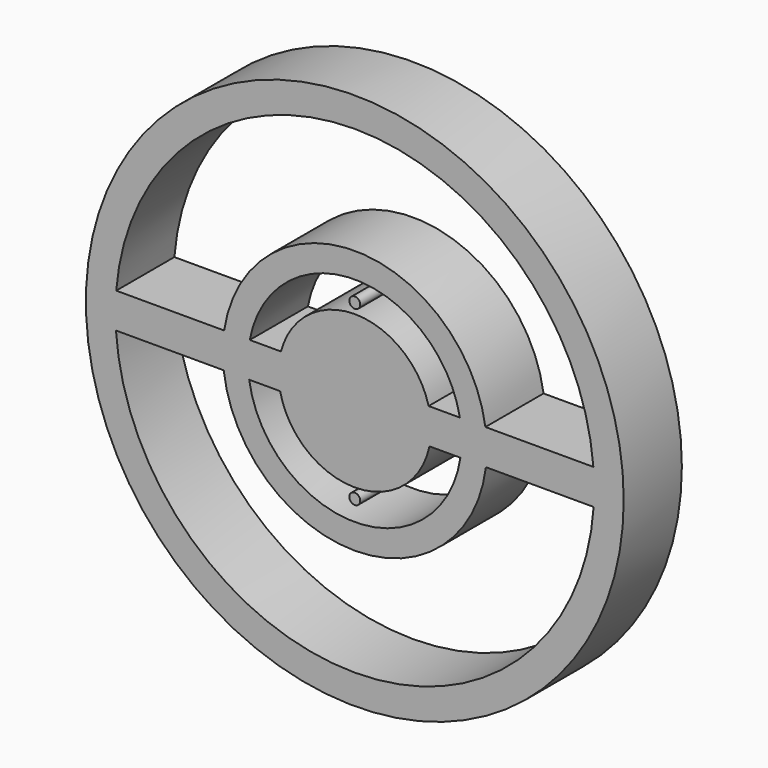
from build123d import *

# Parameters (mm, degrees)
F0_R     = 93.98
F0_W     = 9.525
F0_H     = 25.4
F1_DEPTH = 25.4
F0_R_2   = 1.905


# Not quite as in the source:
# - a feature of the source that left no trace in its solid (it failed there, or was rolled back) is left out


with BuildPart() as f1:
    # F0 (on Front) → F1 (new body)
    with BuildSketch(Plane.XZ):
        Circle(F0_R)
        with BuildLine():
            ThreePointArc((-45.8102837042, -5.5278504869), (0, -46.1425966333), (45.8102837042, -5.5278504869))
            Line((45.8102837042, -5.5278504869), (83.4638586571, -5.5278504869))
            ThreePointArc((83.4638586571, -5.5278504869), (0, -83.646714418), (-83.4638586571, -5.5278504869))
            Line((-83.4638586571, -5.5278504869), (-45.8102837042, -5.5278504869))
        make_face(mode=Mode.SUBTRACT)
        with BuildLine():
            ThreePointArc((36.9132450635, -5.5278504869), (0, -37.3248548841), (-36.9132450635, -5.5278504869))
            Line((-36.9132450635, -5.5278504869), (-26.090836878, -5.5278504869))
            ThreePointArc((-26.090836878, -5.5278504869), (0, -26.67), (26.090836878, -5.5278504869))
            Line((26.090836878, -5.5278504869), (36.9132450635, -5.5278504869))
        make_face(mode=Mode.SUBTRACT)
        Rectangle(F0_W, F0_H, mode=Mode.SUBTRACT)
        with BuildLine():
            ThreePointArc((-36.7071338058, 6.7624788271), (0, 37.3248548841), (36.7071338058, 6.7624788271))
            Line((36.7071338058, 6.7624788271), (25.7984065421, 6.7624788271))
            ThreePointArc((25.7984065421, 6.7624788271), (0, 26.67), (-25.7984065421, 6.7624788271))
            Line((-25.7984065421, 6.7624788271), (-36.7071338058, 6.7624788271))
        make_face(mode=Mode.SUBTRACT)
        with BuildLine():
            Line((83.3729075482, 6.7624788271), (45.644365525, 6.7624788271))
            ThreePointArc((45.644365525, 6.7624788271), (0, 46.1425966333), (-45.644365525, 6.7624788271))
            Line((-45.644365525, 6.7624788271), (-83.3729075482, 6.7624788271))
            ThreePointArc((-83.3729075482, 6.7624788271), (0, 83.646714418), (83.3729075482, 6.7624788271))
        make_face(mode=Mode.SUBTRACT)
        Rectangle(F0_W, F0_H)
    extrude(amount=F1_DEPTH)


with BuildPart() as f1b:
    # F0 (on Front) → F1, piece 2 (new body)
    with BuildSketch(Plane.XZ):
        with Locations((0, 30.1752)):
            Circle(F0_R_2)
    extrude(amount=F1_DEPTH)


with BuildPart() as f1c:
    # F0 (on Front) → F1, piece 3 (new body)
    with BuildSketch(Plane.XZ):
        with Locations((0, -30.1752)):
            Circle(F0_R_2)
    extrude(amount=F1_DEPTH)


solid = Compound([f1.part, f1b.part, f1c.part])
